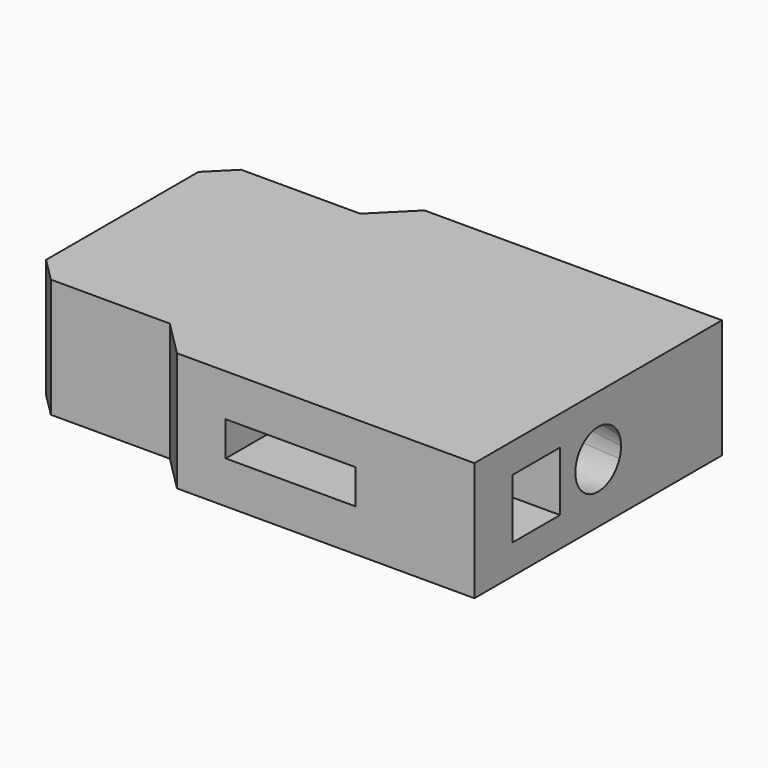
from build123d import *

# Parameters (mm, degrees)
F0_W        = 10
F0_H        = 20
F1_DEPTH    = 10
F3_DEPTH    = 5
F4_T4_DEPTH = 35.7168298797
F4_T9_DEPTH = 35.7168298797
F5_SIZE     = 2
F7_DEPTH    = 26
F9_DEPTH    = 10
F9_TAPER    = -10
F11_DEPTH   = 5
F12_DEPTH   = 9
F13_R       = 1
F14_W       = 4
F14_H       = 8
F15_DEPTH   = 1
F16_SIZE    = 0.99999
F17_DEPTH   = 5


# Not quite as in the source:
# - a fillet or chamfer that OpenCascade refuses, or shapes differently, is made with other operations: its cross-section is extruded or revolved along the edge and cut away or added
# - a fillet or chamfer is up to 0.001 mm smaller than in the source, because OpenCascade refuses the exact size
# - a feature names something its author has since deleted; it is built from what else it names


with BuildPart() as f1:
    # F0 (on Top) → F1 (new body)
    with BuildSketch(Plane.XY):
        with Locations((-7.7272727273, 0)):
            Rectangle(F0_W, F0_H)
        Polygon((-2.7272727273, 13), (-2.7272727273, 10), (-2.7272727273, -10), (-2.7272727273, -13), (27.2727272727, -13), (27.2727272727, 13), align=None)
    extrude(amount=F1_DEPTH)

    # F2 (on face) → F3 (cut)
    with BuildSketch(Plane(origin=(-12.7272727273, 0, 0), x_dir=(0, -1, 0), z_dir=(-1, 0, 0))):
        Polygon((0, 5), (-2.7, 6.35), (-5.35, 6.35), (-5.35, 3.65), (-2.7, 3.65), align=None)
        Polygon((2.7, 3.65), (0, 5), (-2.7, 3.65), align=None)
        Polygon((2.7, 6.35), (0, 5), (2.7, 3.65), (5.35, 3.65), (5.35, 6.35), align=None)
        Polygon((2.7, 6.35), (-2.7, 6.35), (0, 5), align=None)
    extrude(amount=-F3_DEPTH, mode=Mode.SUBTRACT)

    # F4: chamfer of 5 on 2 edges, made by hand


with BuildPart() as f4_tool2:
    # F4_s3 → F4_t4 (new body)
    with BuildSketch(Plane.XY.offset(-12.8584149398)):
        Polygon((2.2727272727, 13), (-2.7272727273, 8), (-2.7272727273, 13), align=None)
    extrude(amount=F4_T4_DEPTH)

    split(bisect_by=Plane.XZ.offset(-10), keep=Keep.BOTTOM)


with BuildPart() as f1_1:
    add(f1.part)

    # F4_t1: cut F4_tool2
    add(f4_tool2.part, mode=Mode.SUBTRACT)


with BuildPart() as f4_tool7:
    # F4_s8 → F4_t9 (new body)
    with BuildSketch(Plane.XY.offset(-12.8584149398)):
        Polygon((-2.7272727273, -8), (2.2727272727, -13), (-2.7272727273, -13), align=None)
    extrude(amount=F4_T9_DEPTH)

    split(bisect_by=Plane.XZ.offset(10), keep=Keep.TOP)


with BuildPart() as f1_2:
    add(f1_1.part)

    # F4_t6: cut F4_tool7
    add(f4_tool7.part, mode=Mode.SUBTRACT)

    # F5
    f5_edges = [f1_2.edges().sort_by_distance(p)[0] for p in [
        (-12.727273, 10, 5),
        (-12.727273, -10, 5),
    ]]
    chamfer(f5_edges, length=F5_SIZE)

    # F6 (on face) → F7 (cut, through all)
    with BuildSketch(Plane(origin=(0, 13, 0), x_dir=(-1, 0, 0), z_dir=(0, 1, 0))):
        Polygon((-14.7727272727, 5), (-17.2727272727, 6), (-17.2727272727, 5), align=None)
        Polygon((-17.2727272727, 6.45), (-17.2727272727, 6), (-14.7727272727, 5), (-11.1477272727, 6.45), align=None)
        Polygon((-11.1477272727, 6.45), (-14.7727272727, 5), (-6.3727272727, 5), (-6.3727272727, 6.45), align=None)
        Polygon((-17.2727272727, 4), (-14.7727272727, 5), (-17.2727272727, 5), align=None)
        Polygon((-11.1477272727, 3.55), (-14.7727272727, 5), (-17.2727272727, 4), (-17.2727272727, 3.55), align=None)
        Polygon((-6.3727272727, 5), (-14.7727272727, 5), (-11.1477272727, 3.55), (-6.3727272727, 3.55), align=None)
    extrude(amount=-F7_DEPTH, mode=Mode.SUBTRACT)

    # F8 (on face) → F9 (cut, through all)
    with BuildSketch(Plane.YZ.offset(27.2727272727)):
        with BuildLine():
            Line((-2.4, 5), (0, 5))
            Line((0, 5), (-2.2400294549, 5.8615497903))
            ThreePointArc((-2.2400294549, 5.8615497903), (-2.3596684822, 5.4381377114), (-2.4, 5))
        make_face()
        with BuildLine():
            Line((-2.2400294549, 5.8615497903), (0, 5))
            Line((0, 5), (2.2400294549, 5.8615497903))
            ThreePointArc((2.2400294549, 5.8615497903), (0, 7.4), (-2.2400294549, 5.8615497903))
        make_face()
        with BuildLine():
            Line((0, 5), (2.2400294549, 4.1384502097))
            ThreePointArc((2.2400294549, 4.1384502097), (2.3596684822, 4.5618622886), (2.4, 5))
            ThreePointArc((2.4, 5), (2.3596684822, 5.4381377114), (2.2400294549, 5.8615497903))
            Line((2.2400294549, 5.8615497903), (0, 5))
        make_face()
        with BuildLine():
            ThreePointArc((-2.2400294549, 4.1384502097), (0, 2.6), (2.2400294549, 4.1384502097))
            Line((2.2400294549, 4.1384502097), (0, 5))
            Line((0, 5), (-2.2400294549, 4.1384502097))
        make_face()
        with BuildLine():
            Line((-2.2400294549, 4.1384502097), (0, 5))
            Line((0, 5), (-2.4, 5))
            ThreePointArc((-2.4, 5), (-2.3596684822, 4.5618622886), (-2.2400294549, 4.1384502097))
        make_face()
    extrude(amount=-F9_DEPTH, taper=F9_TAPER, mode=Mode.SUBTRACT)

    # F10 (on face) → F11 (cut)
    with BuildSketch(Plane(origin=(0, 0, 0), x_dir=(1, 0, 0), z_dir=(0, 0, -1))):
        Polygon((18.2727272727, -3), (18.2727272727, 3), (16.2727272727, 3), (8.2727272727, 3), (8.2727272727, -3), (16.2727272727, -3), align=None)
    extrude(amount=-F11_DEPTH, mode=Mode.SUBTRACT)

    # F12 (cut, through all): faces of the model
    f12_faces = [f1_2.faces().sort_by_distance(p)[0] for p in [
        (17.2727272727, 3.3247194786, 3.0369278497),
        (17.2727272727, -3.3247194786, 3.0369278497),
    ]]
    extrude(f12_faces, amount=-F12_DEPTH, mode=Mode.SUBTRACT)

    # F13
    f13_edges = [f1_2.edges().sort_by_distance(p)[0] for p in [
        (18.272727, -3, 1.187016),
        (8.272727, -3, 1.056669),
        (8.272727, 3, 1.056669),
        (18.272727, 3, 1.187016),
    ]]
    fillet(f13_edges, radius=F13_R)

    # F14 (on face) → F15 (cut)
    with BuildSketch(Plane(origin=(0, 0, 0), x_dir=(1, 0, 0), z_dir=(0, 0, -1))):
        Polygon((8.2727272727, 2), (-12.7272727273, 2), (-12.7272727273, -2), (-6.7272727273, -2), (-2.7272727273, -2), (8.2727272727, -2), align=None)
        with Locations((-4.7272727273, -6)):
            Rectangle(F14_W, F14_H)
    extrude(amount=-F15_DEPTH, mode=Mode.SUBTRACT)

    # F16 (size 1 in the source; OpenCascade refuses exactly that, so slightly less here)
    f16_edges = [f1_2.edges().sort_by_distance(p)[0] for p in [
        (-6.727273, 6, 0),
    ]]
    chamfer(f16_edges, length=F16_SIZE)

    # F8 (on face) → F17 (cut)
    with BuildSketch(Plane.YZ.offset(27.2727272727)):
        Polygon((-4, 7.5), (-6.5, 7.5), (-4, 6.5384615385), align=None)
        Polygon((-4, 6.5384615385), (-6.5, 7.5), (-9, 7.5), (-9, 5), (-4, 5), align=None)
        Polygon((-9, 2.5), (-6.5, 2.5), (-4, 3.4615384615), (-4, 5), (-9, 5), align=None)
        Polygon((-4, 3.4615384615), (-6.5, 2.5), (-4, 2.5), align=None)
    extrude(amount=-F17_DEPTH, mode=Mode.SUBTRACT)


solid = f1_2.part
